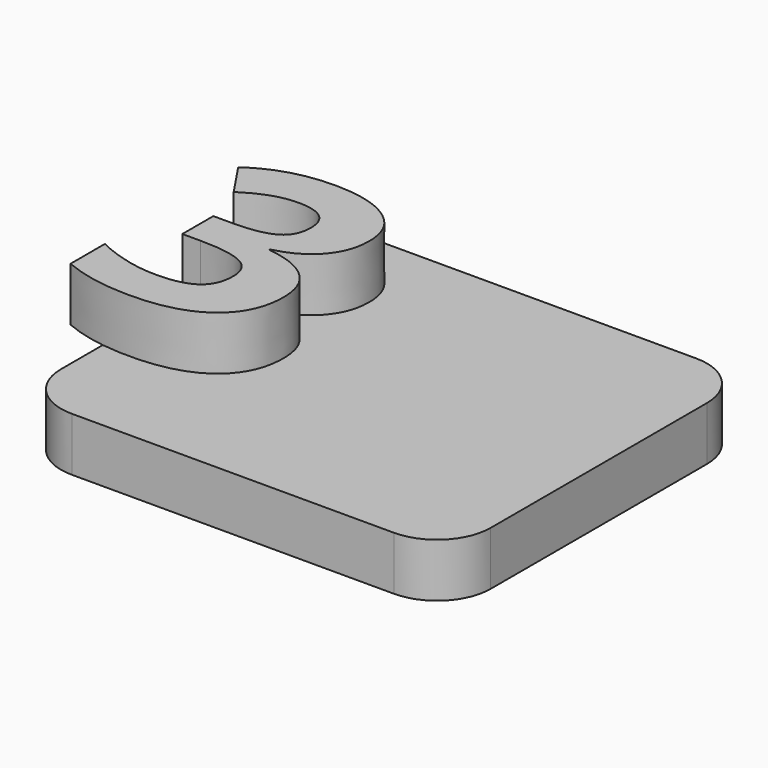
from build123d import *

# Parameters (mm, degrees)
F1_DEPTH     = 6.35
F2_TEXT_SIZE = 39.5590620529
F3_DEPTH     = 6.35


# Not quite as in the source:
# - Text() gives the source's letters only with a copy of the font that has no kerning and outlines rounded to 1/6400 em; it was checked with that copy


with BuildPart() as f1:
    # F0 (on Top) → F1 (new body)
    with BuildSketch(Plane.XY):
        with BuildLine():
            Line((7.4490033254, 55.0096375704), (-30.6509966746, 55.0096375704))
            ThreePointArc((-30.6509966746, 55.0096375704), (-35.1411247351, 53.1497656309), (-37.0009966746, 48.6596375704))
            Line((-37.0009966746, 48.6596375704), (-37.0009966746, 16.7040545493))
            ThreePointArc((-37.0009966746, 16.7040545493), (-35.1411247351, 12.2139264888), (-30.6509966746, 10.3540545493))
            Line((-30.6509966746, 10.3540545493), (7.4490033254, 10.3540545493))
            ThreePointArc((7.4490033254, 10.3540545493), (11.9391313859, 12.2139264888), (13.7990033254, 16.7040545493))
            Line((13.7990033254, 16.7040545493), (13.7990033254, 48.6596375704))
            ThreePointArc((13.7990033254, 48.6596375704), (11.9391313859, 53.1497656309), (7.4490033254, 55.0096375704))
        make_face()
    extrude(amount=F1_DEPTH)

    # F2 (on face) → F3 (join)
    with BuildSketch(Plane.XY.offset(6.35)):
        with Locations((-43.3711186051, 23.0449531227)):
            Text('3', F2_TEXT_SIZE, font='Open Sans', font_style=FontStyle.BOLD, text_align=(TextAlign.LEFT, TextAlign.BOTTOM))
    extrude(amount=F3_DEPTH)


solid = f1.part
